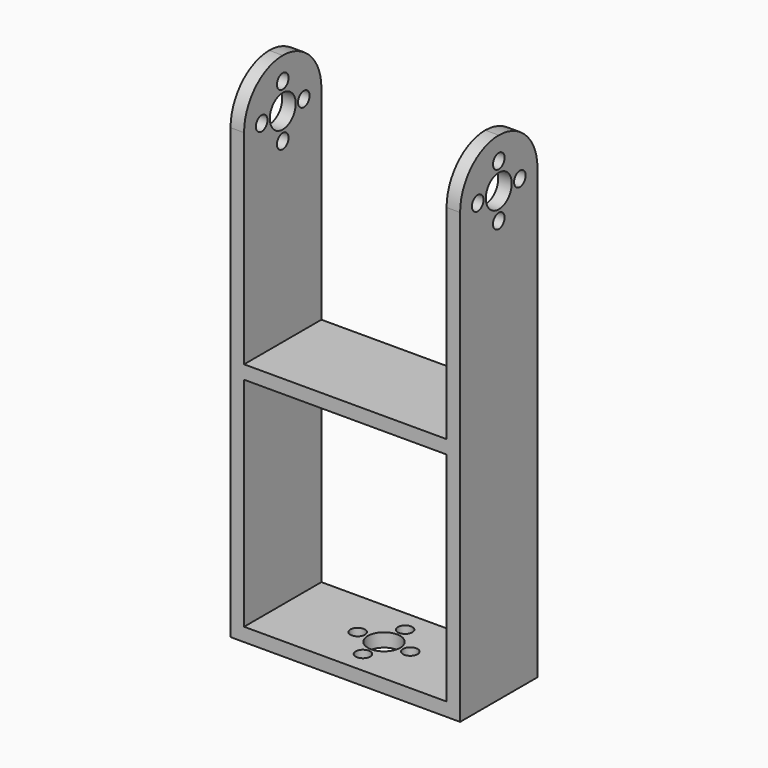
from build123d import *

# Parameters (mm, degrees)
F0_W      = 60.325
F0_H      = 25.4
F1_DEPTH  = 3.556
F2_W      = 3.556
F2_H      = 25.4
F3_DEPTH  = 127
F4_R      = 12.7
F5_R      = 12.69999
F6_R      = 4.2545
F6_R_2    = 1.905
F7_DEPTH  = 254
F8_R      = 4.2545
F8_R_2    = 1.905
F9_DEPTH  = 25.4
F10_W     = 25.4
F10_H     = 3.556
F11_DEPTH = 53.34


# Not quite as in the source:
# - a fillet or chamfer is up to 0.001 mm smaller than in the source, because OpenCascade refuses the exact size


with BuildPart() as f1:
    # F0 (on Top) → F1 (new body)
    with BuildSketch(Plane.XY):
        with Locations((3.8735, 0)):
            Rectangle(F0_W, F0_H)
    extrude(amount=F1_DEPTH)

    # F2 (on face) → F3 (join)
    with BuildSketch(Plane.XY.offset(3.556)):
        with Locations((-24.511, 0)):
            Rectangle(F2_W, F2_H)
        with Locations((32.258, 0)):
            Rectangle(F2_W, F2_H)
    extrude(amount=F3_DEPTH)

    # F4
    f4_edges = [f1.edges().sort_by_distance(p)[0] for p in [
        (32.258, 12.7, 130.556),
    ]]
    fillet(f4_edges, radius=F4_R)

    # F5 (radius 12.7 in the source; OpenCascade refuses exactly that, so slightly less here)
    f5_edges = [f1.edges().sort_by_distance(p)[0] for p in [
        (32.258, -12.7, 130.556),
        (-24.511, -12.7, 130.556),
        (-24.511, 12.7, 130.556),
    ]]
    fillet(f5_edges, radius=F5_R)

    # F6 (on face) → F7 (cut)
    with BuildSketch(Plane.YZ.offset(34.036)):
        with Locations((0, 117.6655)):
            Circle(F6_R)
        with Locations((0, 124.587)):
            Circle(F6_R_2)
        with Locations((-6.9215, 117.6655)):
            Circle(F6_R_2)
        with Locations((0, 110.744)):
            Circle(F6_R_2)
        with Locations((6.9215, 117.6655)):
            Circle(F6_R_2)
    extrude(amount=-F7_DEPTH, mode=Mode.SUBTRACT)

    # F8 (on face) → F9 (cut)
    with BuildSketch(Plane.XY.offset(3.556)):
        with Locations((3.8735, 0)):
            Circle(F8_R)
        with Locations((-3.048, 0)):
            Circle(F8_R_2)
        with Locations((3.8735, 6.9215)):
            Circle(F8_R_2)
        with Locations((3.8735, -6.9215)):
            Circle(F8_R_2)
        with Locations((10.795, 0)):
            Circle(F8_R_2)
    extrude(amount=-F9_DEPTH, mode=Mode.SUBTRACT)

    # F10 (on face) → F11 (join)
    with BuildSketch(Plane.YZ.offset(-22.733)):
        with Locations((0, 62.484)):
            Rectangle(F10_W, F10_H)
    extrude(amount=F11_DEPTH)


solid = f1.part
